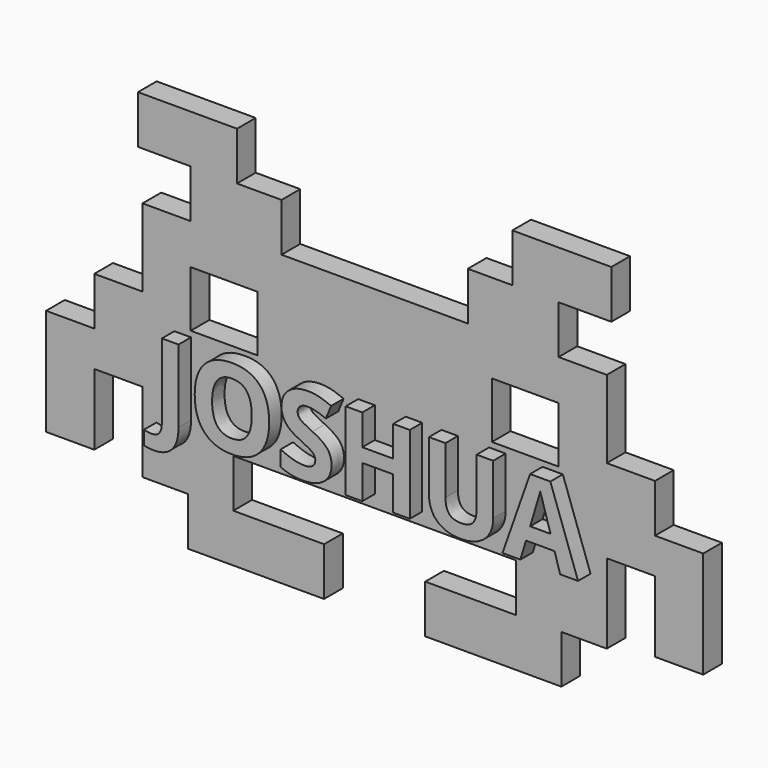
from build123d import *

# Parameters (mm, degrees)
F1_TEXT_SIZE = 35.7067348766
F2_DEPTH     = 5.08
F0_DEPTH     = 7.62


# Not quite as in the source:
# - Text() gives the source's letters only with a copy of the font that has no kerning and outlines rounded to 1/6400 em; it was checked with that copy


with BuildPart() as f2:
    # F1 (on Front) → F2 (new body)
    with BuildSketch(Plane.XZ):
        with Locations((-24.2589620852, -15.119778458)):
            Text('JOSHUA', F1_TEXT_SIZE, font='Open Sans', font_style=FontStyle.BOLD, text_align=(TextAlign.LEFT, TextAlign.BOTTOM))
    extrude(amount=F2_DEPTH)

    # F1 (on Front) → F0 (join)
    with BuildSketch(Plane.XZ):
        Polygon((-15.7191818841, 43.678149581), (-31.4383637682, 43.678149581), (-31.4383637682, 18.3543078785), (-31.4383637682, 3.0076354742), (-31.4383637682, -8.9530429808), (-31.4383637682, -34.8967627195), (-16.6428352279, -34.8967627195), (-1.8473066877, -34.8967627195), (-1.8473066877, -19.1775808354), (44.23101875, -19.1775808354), (90.3093441877, -19.1775808354), (90.3093441877, -34.8967627195), (105.1048727279, -34.8967627195), (119.9004012682, -34.8967627195), (119.9004012682, -8.9530429808), (119.9004012682, -2.2653539024), (119.9004012682, 18.3543078785), (119.9004012682, 43.678149581), (104.1812193841, 43.678149581), (74.5901623036, 43.678149581), (13.8718751964, 43.678149581), align=None)
        with BuildLine():
            add(Edge.make_bspline(
                [(-17.6839016083, -20.2805174832), (-19.7230909204, -22.6181927821), (-23.7177818847, -22.6181927821)],
                knots=[0, 0, 0, 1, 1, 1], degree=2))
            add(Edge.make_bspline(
                [(-23.7177818847, -22.6181927821), (-25.5477520472, -22.6181927821), (-26.9090713143, -22.2332295467)],
                knots=[0, 0, 0, 1, 1, 1], degree=2))
            Line((-26.9090713143, -22.2332295467), (-26.9090713143, -17.7364126232))
            add(Edge.make_bspline(
                [(-26.9090713143, -17.7364126232), (-25.5142769832, -18.0823216173), (-24.3649664544, -18.0823216173)],
                knots=[0, 0, 0, 1, 1, 1], degree=2))
            add(Edge.make_bspline(
                [(-24.3649664544, -18.0823216173), (-22.5852088879, -18.0823216173), (-21.8180720058, -16.9748549184)],
                knots=[0, 0, 0, 1, 1, 1], degree=2))
            add(Edge.make_bspline(
                [(-21.8180720058, -16.9748549184), (-21.0509351236, -15.8673882195), (-21.0509351236, -13.5129753886)],
                knots=[0, 0, 0, 1, 1, 1], degree=2))
            Line((-21.0509351236, -13.5129753886), (-21.0509351236, 10.3714827375))
            Line((-21.0509351236, 10.3714827375), (-15.6447122962, 10.3714827375))
            Line((-15.6447122962, 10.3714827375), (-15.6447122962, -13.4795003246))
            add(Edge.make_bspline(
                [(-15.6447122962, -13.4795003246), (-15.6447122962, -17.9428421842), (-17.6839016083, -20.2805174832)],
                knots=[0, 0, 0, 1, 1, 1], degree=2))
        make_face(mode=Mode.SUBTRACT)
        with BuildLine():
            add(Edge.make_bspline(
                [(10.7950090444, 7.3894124576), (13.9081899915, 4.0056414103), (13.9081899915, -2.3378832077)],
                knots=[0, 0, 0, 1, 1, 1], degree=2))
            add(Edge.make_bspline(
                [(13.9081899915, -2.3378832077), (13.9081899915, -8.6702494709), (10.7699027465, -12.0707580502)],
                knots=[0, 0, 0, 1, 1, 1], degree=2))
            add(Edge.make_bspline(
                [(10.7699027465, -12.0707580502), (7.6316155015, -15.4712666295), (1.7734793108, -15.4712666295)],
                knots=[0, 0, 0, 1, 1, 1], degree=2))
            add(Edge.make_bspline(
                [(1.7734793108, -15.4712666295), (-4.0846568799, -15.4712666295), (-7.2229441249, -12.0707580502)],
                knots=[0, 0, 0, 1, 1, 1], degree=2))
            add(Edge.make_bspline(
                [(-7.2229441249, -12.0707580502), (-10.36123137, -8.6702494709), (-10.36123137, -2.3044081437)],
                knots=[0, 0, 0, 1, 1, 1], degree=2))
            add(Edge.make_bspline(
                [(-10.36123137, -2.3044081437), (-10.36123137, 4.0614331835), (-7.214575359, 7.4173083442)],
                knots=[0, 0, 0, 1, 1, 1], degree=2))
            add(Edge.make_bspline(
                [(-7.214575359, 7.4173083442), (-4.067919348, 10.7731835048), (1.8069543747, 10.7731835048)],
                knots=[0, 0, 0, 1, 1, 1], degree=2))
            add(Edge.make_bspline(
                [(1.8069543747, 10.7731835048), (7.6818280974, 10.7731835048), (10.7950090444, 7.3894124576)],
                knots=[0, 0, 0, 1, 1, 1], degree=2))
        make_face(mode=Mode.SUBTRACT)
        with BuildLine():
            add(Edge.make_bspline(
                [(32.9136575473, -3.830313142), (34.2387121619, -5.5459101692), (34.2387121619, -8.0398024333)],
                knots=[0, 0, 0, 1, 1, 1], degree=2))
            add(Edge.make_bspline(
                [(34.2387121619, -8.0398024333), (34.2387121619, -11.4933131971), (31.7531886638, -13.4822899133)],
                knots=[0, 0, 0, 1, 1, 1], degree=2))
            add(Edge.make_bspline(
                [(31.7531886638, -13.4822899133), (29.2676651658, -15.4712666295), (24.8433775475, -15.4712666295)],
                knots=[0, 0, 0, 1, 1, 1], degree=2))
            add(Edge.make_bspline(
                [(24.8433775475, -15.4712666295), (20.7594197459, -15.4712666295), (17.6239220896, -13.9314136879)],
                knots=[0, 0, 0, 1, 1, 1], degree=2))
            Line((17.6239220896, -13.9314136879), (17.6239220896, -8.9101540959))
            add(Edge.make_bspline(
                [(17.6239220896, -8.9101540959), (20.2015020135, -10.0650438021), (21.989628346, -10.5336946973)],
                knots=[0, 0, 0, 1, 1, 1], degree=2))
            add(Edge.make_bspline(
                [(21.989628346, -10.5336946973), (23.7777546785, -11.0023455926), (25.2618158468, -11.0023455926)],
                knots=[0, 0, 0, 1, 1, 1], degree=2))
            add(Edge.make_bspline(
                [(25.2618158468, -11.0023455926), (27.035994236, -11.0023455926), (27.9872439698, -10.3244755476)],
                knots=[0, 0, 0, 1, 1, 1], degree=2))
            add(Edge.make_bspline(
                [(27.9872439698, -10.3244755476), (28.9384937036, -9.6466055027), (28.9384937036, -8.3020237675)],
                knots=[0, 0, 0, 1, 1, 1], degree=2))
            add(Edge.make_bspline(
                [(28.9384937036, -8.3020237675), (28.9384937036, -7.554414006), (28.5200554043, -6.968600387)],
                knots=[0, 0, 0, 1, 1, 1], degree=2))
            add(Edge.make_bspline(
                [(28.5200554043, -6.968600387), (28.1016171049, -6.3827867679), (27.2898468042, -5.8443961561)],
                knots=[0, 0, 0, 1, 1, 1], degree=2))
            add(Edge.make_bspline(
                [(27.2898468042, -5.8443961561), (26.4780765035, -5.3060055443), (23.9841842395, -4.1176407742)],
                knots=[0, 0, 0, 1, 1, 1], degree=2))
            add(Edge.make_bspline(
                [(23.9841842395, -4.1176407742), (21.6520881179, -3.0185428412), (20.4832504684, -2.0087117455)],
                knots=[0, 0, 0, 1, 1, 1], degree=2))
            add(Edge.make_bspline(
                [(20.4832504684, -2.0087117455), (19.3144128189, -0.9988806498), (18.6170156533, 0.3457010854)],
                knots=[0, 0, 0, 1, 1, 1], degree=2))
            add(Edge.make_bspline(
                [(18.6170156533, 0.3457010854), (17.9196184878, 1.6902828206), (17.9196184878, 3.4811987418)],
                knots=[0, 0, 0, 1, 1, 1], degree=2))
            add(Edge.make_bspline(
                [(17.9196184878, 3.4811987418), (17.9196184878, 6.8677593777), (20.2126603681, 8.8009443206)],
                knots=[0, 0, 0, 1, 1, 1], degree=2))
            add(Edge.make_bspline(
                [(20.2126603681, 8.8009443206), (22.5057022485, 10.7341292636), (26.5506058087, 10.7341292636)],
                knots=[0, 0, 0, 1, 1, 1], degree=2))
            add(Edge.make_bspline(
                [(26.5506058087, 10.7341292636), (28.5367929363, 10.7341292636), (30.3416568007, 10.2654783683)],
                knots=[0, 0, 0, 1, 1, 1], degree=2))
            add(Edge.make_bspline(
                [(30.3416568007, 10.2654783683), (32.1465206652, 9.7968274731), (34.1159702607, 8.9432133424)],
                knots=[0, 0, 0, 1, 1, 1], degree=2))
            Line((34.1159702607, 8.9432133424), (32.3752669355, 4.7365136398))
            add(Edge.make_bspline(
                [(32.3752669355, 4.7365136398), (30.3332880347, 5.5733902384), (28.9998646542, 5.9053512892)],
                knots=[0, 0, 0, 1, 1, 1], degree=2))
            add(Edge.make_bspline(
                [(28.9998646542, 5.9053512892), (27.6664412736, 6.23731234), (26.3776513117, 6.23731234)],
                knots=[0, 0, 0, 1, 1, 1], degree=2))
            add(Edge.make_bspline(
                [(26.3776513117, 6.23731234), (24.8433775475, 6.23731234), (24.0232384808, 5.5231776425)],
                knots=[0, 0, 0, 1, 1, 1], degree=2))
            add(Edge.make_bspline(
                [(24.0232384808, 5.5231776425), (23.2030994141, 4.809042945), (23.2030994141, 3.6597324161)],
                knots=[0, 0, 0, 1, 1, 1], degree=2))
            add(Edge.make_bspline(
                [(23.2030994141, 3.6597324161), (23.2030994141, 2.9455977186), (23.5350604649, 2.4127862841)],
                knots=[0, 0, 0, 1, 1, 1], degree=2))
            add(Edge.make_bspline(
                [(23.5350604649, 2.4127862841), (23.8670215157, 1.8799748496), (24.5895249792, 1.3834280678)],
                knots=[0, 0, 0, 1, 1, 1], degree=2))
            add(Edge.make_bspline(
                [(24.5895249792, 1.3834280678), (25.3120284427, 0.8868812859), (28.0123502678, -0.4019086761)],
                knots=[0, 0, 0, 1, 1, 1], degree=2))
            add(Edge.make_bspline(
                [(28.0123502678, -0.4019086761), (31.5886029327, -2.1147161147), (32.9136575473, -3.830313142)],
                knots=[0, 0, 0, 1, 1, 1], degree=2))
        make_face(mode=Mode.SUBTRACT)
        Polygon((59.7467108894, 10.3714827375), (59.7467108894, -15.119778458), (54.3572255939, -15.119778458), (54.3572255939, -4.1176407742), (44.2644938139, -4.1176407742), (44.2644938139, -15.119778458), (38.8582709865, -15.119778458), (38.8582709865, 10.3714827375), (44.2644938139, 10.3714827375), (44.2644938139, 0.3791761494), (54.3572255939, 0.3791761494), (54.3572255939, 10.3714827375), align=None, mode=Mode.SUBTRACT)
        with BuildLine():
            Line((81.5389775187, 10.3714827375), (86.9284628142, 10.3714827375))
            Line((86.9284628142, 10.3714827375), (86.9284628142, -6.1205654337))
            add(Edge.make_bspline(
                [(86.9284628142, -6.1205654337), (86.9284628142, -8.9492083372), (85.6647791502, -11.0748748978)],
                knots=[0, 0, 0, 1, 1, 1], degree=2))
            add(Edge.make_bspline(
                [(85.6647791502, -11.0748748978), (84.4010954862, -13.2005414584), (82.0104180027, -14.3359040439)],
                knots=[0, 0, 0, 1, 1, 1], degree=2))
            add(Edge.make_bspline(
                [(82.0104180027, -14.3359040439), (79.6197405191, -15.4712666295), (76.3615009616, -15.4712666295)],
                knots=[0, 0, 0, 1, 1, 1], degree=2))
            add(Edge.make_bspline(
                [(76.3615009616, -15.4712666295), (71.4462457388, -15.4712666295), (68.7263967931, -12.9494784788)],
                knots=[0, 0, 0, 1, 1, 1], degree=2))
            add(Edge.make_bspline(
                [(68.7263967931, -12.9494784788), (66.0065478474, -10.4276903281), (66.0065478474, -6.0536153058)],
                knots=[0, 0, 0, 1, 1, 1], degree=2))
            Line((66.0065478474, -6.0536153058), (66.0065478474, 10.3714827375))
            Line((66.0065478474, 10.3714827375), (71.3904539655, 10.3714827375))
            Line((71.3904539655, 10.3714827375), (71.3904539655, -5.2334762391))
            add(Edge.make_bspline(
                [(71.3904539655, -5.2334762391), (71.3904539655, -8.1792818664), (72.576029147, -9.5573386655)],
                knots=[0, 0, 0, 1, 1, 1], degree=2))
            add(Edge.make_bspline(
                [(72.576029147, -9.5573386655), (73.7616043284, -10.9353954647), (76.5009803947, -10.9353954647)],
                knots=[0, 0, 0, 1, 1, 1], degree=2))
            add(Edge.make_bspline(
                [(76.5009803947, -10.9353954647), (79.1510896239, -10.9353954647), (80.3450335713, -9.5489698995)],
                knots=[0, 0, 0, 1, 1, 1], degree=2))
            add(Edge.make_bspline(
                [(80.3450335713, -9.5489698995), (81.5389775187, -8.1625443344), (81.5389775187, -5.2000011751)],
                knots=[0, 0, 0, 1, 1, 1], degree=2))
            Line((81.5389775187, -5.2000011751), (81.5389775187, 10.3714827375))
        make_face(mode=Mode.SUBTRACT)
        Polygon((114.6011823436, -15.119778458), (108.7765212168, -15.119778458), (106.9298135224, -9.049633529), (97.6349040998, -9.049633529), (95.7881964054, -15.119778458), (89.9635352787, -15.119778458), (98.9627483031, 10.4774871066), (105.5684942552, 10.4774871066), align=None, mode=Mode.SUBTRACT)
        Polygon((-15.7191818841, 12.2397858128), (-15.7191818841, 27.9589676969), (-15.7191818841, 30.4893627763), (6.0166767798, 30.4893627763), (6.0166767798, 12.2397858128), (0, 12.2397858128), align=None, mode=Mode.SUBTRACT)
        Polygon((104.1812193841, 30.4893627763), (104.1812193841, 27.9589676969), (104.1812193841, 12.2397858128), (88.4620375, 12.2397858128), (82.4453607202, 12.2397858128), (82.4453607202, 30.4893627763), align=None, mode=Mode.SUBTRACT)
        Polygon((135.6195831522, 18.3543078785), (119.9004012682, 18.3543078785), (119.9004012682, -2.2653539024), (119.9004012682, -8.9530429808), (135.6195831522, -8.9530429808), (135.6195831522, -32.129380931), (151.3387650363, -32.129380931), (151.3387650363, -20.5412119559), (151.3387650363, -8.9530429808), (151.3387650363, 2.6351259944), (135.6195831522, 2.6351259944), align=None)
        Polygon((-31.4383637682, 3.0076354742), (-31.4383637682, 18.3543078785), (-47.1575456522, 18.3543078785), (-47.1575456522, 2.6351259944), (-62.8767275363, 2.6351259944), (-62.8767275363, -8.9530429808), (-62.8767275363, -20.5412119559), (-62.8767275363, -32.129380931), (-47.1575456522, -32.129380931), (-47.1575456522, -8.9530429808), (-31.4383637682, -8.9530429808), align=None)
        Polygon((105.1048727279, -50.6159446036), (105.1048727279, -34.8967627195), (90.3093441877, -34.8967627195), (60.7182871072, -34.8967627195), (60.7182871072, -50.6159446036), align=None)
        Polygon((-1.8473066877, -34.8967627195), (-16.6428352279, -34.8967627195), (-16.6428352279, -50.6159446036), (27.7437503928, -50.6159446036), (27.7437503928, -34.8967627195), align=None)
        Polygon((-32.9294079892, 59.397331465), (-15.7191818841, 59.397331465), (-0.6430769316, 59.397331465), (-0.6430769316, 75.1165133491), (-32.9294079892, 75.1165133491), align=None)
        Polygon((89.1051144316, 75.1165133491), (89.1051144316, 59.397331465), (104.1812193841, 59.397331465), (121.3914454892, 59.397331465), (121.3914454892, 75.1165133491), align=None)
        Polygon((-15.7191818841, 59.397331465), (-15.7191818841, 43.678149581), (13.8718751964, 43.678149581), (13.8718751964, 59.397331465), (-0.6430769316, 59.397331465), align=None)
        Polygon((74.5901623036, 59.397331465), (74.5901623036, 43.678149581), (104.1812193841, 43.678149581), (104.1812193841, 59.397331465), (89.1051144316, 59.397331465), align=None)
        with Locations((-24.2589620852, -15.119778458)):
            Text('JOSHUA', F1_TEXT_SIZE, font='Open Sans', font_style=FontStyle.BOLD, text_align=(TextAlign.LEFT, TextAlign.BOTTOM))
        with BuildLine():
            add(Edge.make_bspline(
                [(-3.0552986636, 4.1004874248), (-4.6927872083, 1.9301874456), (-4.6927872083, -2.3378832077)],
                knots=[0, 0, 0, 1, 1, 1], degree=2))
            add(Edge.make_bspline(
                [(-4.6927872083, -2.3378832077), (-4.6927872083, -6.6115330382), (-3.0720361955, -8.7734642514)],
                knots=[0, 0, 0, 1, 1, 1], degree=2))
            add(Edge.make_bspline(
                [(-3.0720361955, -8.7734642514), (-1.4512851828, -10.9353954647), (1.7734793108, -10.9353954647)],
                knots=[0, 0, 0, 1, 1, 1], degree=2))
            add(Edge.make_bspline(
                [(1.7734793108, -10.9353954647), (8.2397458298, -10.9353954647), (8.2397458298, -2.3378832077)],
                knots=[0, 0, 0, 1, 1, 1], degree=2))
            add(Edge.make_bspline(
                [(8.2397458298, -2.3378832077), (8.2397458298, 6.270787404), (1.8069543747, 6.270787404)],
                knots=[0, 0, 0, 1, 1, 1], degree=2))
            add(Edge.make_bspline(
                [(1.8069543747, 6.270787404), (-1.4178101188, 6.270787404), (-3.0552986636, 4.1004874248)],
                knots=[0, 0, 0, 1, 1, 1], degree=2))
        make_face()
        with BuildLine():
            Line((98.996223367, -4.5193415415), (105.6354443831, -4.5193415415))
            add(Edge.make_bspline(
                [(105.6354443831, -4.5193415415), (103.0746019912, 3.726682544), (102.7510097064, 4.809042945)],
                knots=[0, 0, 0, 1, 1, 1], degree=2))
            add(Edge.make_bspline(
                [(102.7510097064, 4.809042945), (102.4274174216, 5.8914033459), (102.2879379884, 6.5162712063)],
                knots=[0, 0, 0, 1, 1, 1], degree=2))
            add(Edge.make_bspline(
                [(102.2879379884, 6.5162712063), (101.713282724, 4.2846002765), (98.996223367, -4.5193415415)],
                knots=[0, 0, 0, 1, 1, 1], degree=2))
        make_face()
    extrude(amount=-F0_DEPTH)


solid = f2.part
